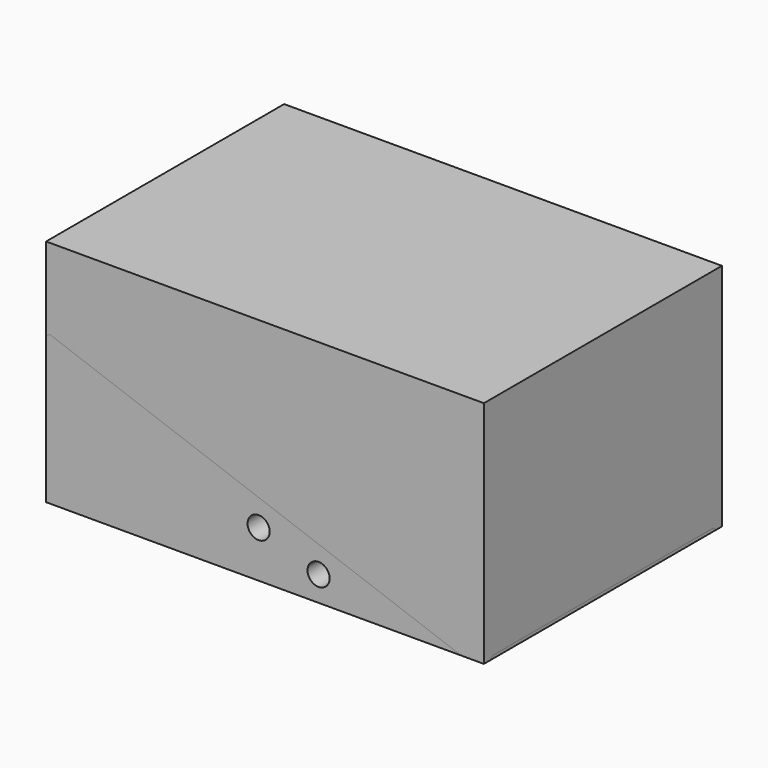
from build123d import *

# Parameters (mm, degrees)
F1_DEPTH      = 35
F1_DEPTH_BACK = 35
F14_W         = 103
F14_H         = 70
F15_DEPTH     = 54
F16_T1_DEPTH  = 122.3961453181
F16_T3_DEPTH  = 88.1090116667
F19_START     = 30
F19_DEPTH     = 5
F20_START     = -30
F20_DEPTH     = 5
F21_R         = 2.6
F22_DEPTH     = 5


# Not quite as in the source:
# - a fillet or chamfer that OpenCascade refuses, or shapes differently, is made with other operations: its cross-section is extruded or revolved along the edge and cut away or added
# - a feature names something its author has since deleted; it is built from what else it names


with BuildPart() as f1:
    # F0 (on Front) → F1 (new body, two sides)
    with BuildSketch(Plane.XZ) as f1_sk:
        Polygon((0, 38), (0, 0), (103, 0), (103, 0.7238095238), align=None)
    extrude(amount=F1_DEPTH)
    extrude(f1_sk.sketch, amount=-F1_DEPTH_BACK)

    # F3 (on offset) → F4 (revolve, cut)
    with BuildSketch(Plane(origin=(12.1597561954, 0, 33.5993263293), x_dir=(0.9403152653, 0, -0.3403045722), z_dir=(0.3403045722, 0, 0.9403152653))):
        with BuildLine():
            ThreePointArc((-3.1315737436, 0), (22.0684262564, -25.2), (47.2684262564, 0))
            Line((47.2684262564, 0), (-3.1315737436, 0))
        make_face()
    revolve(axis=Axis((32.9110342852, 0, 26.089339973), (0.9403152653, 0, -0.3403045722)), mode=Mode.SUBTRACT)

    # F3 (on offset) → F5 (revolve, cut)
    with BuildSketch(Plane(origin=(12.1597561954, 0, 33.5993263293), x_dir=(0.9403152653, 0, -0.3403045722), z_dir=(0.3403045722, 0, 0.9403152653))):
        with BuildLine():
            ThreePointArc((56.9684262564, -15), (62.0684262564, -20.1), (67.1684262564, -15))
            Line((67.1684262564, -15), (62.0684262564, -15))
            Line((62.0684262564, -15), (56.9684262564, -15))
        make_face()
    revolve(axis=Axis((68.1258409703, -15, 13.3449337441), (-0.9403152653, 0, 0.3403045722)), mode=Mode.SUBTRACT)

    # F3 (on offset) → F6 (revolve, cut)
    with BuildSketch(Plane(origin=(12.1597561954, 0, 33.5993263293), x_dir=(0.9403152653, 0, -0.3403045722), z_dir=(0.3403045722, 0, 0.9403152653))):
        with BuildLine():
            ThreePointArc((51.8684262564, 15), (62.0684262564, 4.8), (72.2684262564, 15))
            Line((72.2684262564, 15), (62.0684262564, 15))
            Line((62.0684262564, 15), (51.8684262564, 15))
        make_face()
    revolve(axis=Axis((65.7280370438, 15, 14.2127104032), (-0.9403152653, 0, 0.3403045722)), mode=Mode.SUBTRACT)

    # F3 (on offset) → F7 (revolve, cut)
    with BuildSketch(Plane(origin=(12.1597561954, 0, 33.5993263293), x_dir=(0.9403152653, 0, -0.3403045722), z_dir=(0.3403045722, 0, 0.9403152653))):
        with BuildLine():
            ThreePointArc((80.0684262564, -15), (82.0684262564, -17), (84.0684262564, -15))
            Line((84.0684262564, -15), (82.0684262564, -15))
            Line((82.0684262564, -15), (80.0684262564, -15))
        make_face()
    revolve(axis=Axis((88.3896349374, -15, 6.0113702131), (-0.9403152653, 0, 0.3403045722)), mode=Mode.SUBTRACT)

    # F3 (on offset) → F8 (revolve, cut)
    with BuildSketch(Plane(origin=(12.1597561954, 0, 33.5993263293), x_dir=(0.9403152653, 0, -0.3403045722), z_dir=(0.3403045722, 0, 0.9403152653))):
        with BuildLine():
            ThreePointArc((79.4684262564, 15), (82.0684262564, 12.4), (84.6684262564, 15))
            Line((84.6684262564, 15), (82.0684262564, 15))
            Line((82.0684262564, 15), (79.4684262564, 15))
        make_face()
    revolve(axis=Axis((88.1075403578, 15, 6.1134615848), (-0.9403152653, 0, 0.3403045722)), mode=Mode.SUBTRACT)

    # F16: chamfer of 2.5 on 3 edges, made by hand

    # F16_s2 → F16_t1 (cut)
    with BuildSketch(Plane(origin=(96.8857257323, 0, -35.0634055031), x_dir=(0, 1, 0), z_dir=(-0.9403152653, 0, 0.3403045722))):
        Polygon((-32.5, -35.7319800811), (-35, -33.2319800811), (-35, -35.7319800811), align=None)
        Polygon((32.5, -35.7319800811), (35, -33.2319800811), (35, -35.7319800811), align=None)
    extrude(amount=F16_T1_DEPTH, mode=Mode.SUBTRACT)

    # F16_s4 → F16_t3 (cut)
    with BuildSketch(Plane.XZ.offset(-44.0545058334)):
        Polygon((3.3507614305, 36.7873434823), (0, 34.4365553191), (0, 38), align=None)
    extrude(amount=F16_T3_DEPTH, mode=Mode.SUBTRACT)


with BuildPart() as f9:
    # F3 (on offset) → F9 (revolve)
    with BuildSketch(Plane(origin=(12.1597561954, 0, 33.5993263293), x_dir=(0.9403152653, 0, -0.3403045722), z_dir=(0.3403045722, 0, 0.9403152653))):
        with BuildLine():
            ThreePointArc((-3.1315737436, 0), (22.0684262564, -25.2), (47.2684262564, 0))
            Line((47.2684262564, 0), (-3.1315737436, 0))
        make_face()
    revolve(axis=Axis((32.9110342852, 0, 26.089339973), (0.9403152653, 0, -0.3403045722)))


with BuildPart() as f10:
    # F3 (on offset) → F10 (revolve)
    with BuildSketch(Plane(origin=(12.1597561954, 0, 33.5993263293), x_dir=(0.9403152653, 0, -0.3403045722), z_dir=(0.3403045722, 0, 0.9403152653))):
        with BuildLine():
            ThreePointArc((51.8684262564, 15), (62.0684262564, 4.8), (72.2684262564, 15))
            Line((72.2684262564, 15), (62.0684262564, 15))
            Line((62.0684262564, 15), (51.8684262564, 15))
        make_face()
    revolve(axis=Axis((65.7280370438, 15, 14.2127104032), (-0.9403152653, 0, 0.3403045722)))


with BuildPart() as f11:
    # F3 (on offset) → F11 (revolve)
    with BuildSketch(Plane(origin=(12.1597561954, 0, 33.5993263293), x_dir=(0.9403152653, 0, -0.3403045722), z_dir=(0.3403045722, 0, 0.9403152653))):
        with BuildLine():
            ThreePointArc((56.9684262564, -15), (62.0684262564, -20.1), (67.1684262564, -15))
            Line((67.1684262564, -15), (62.0684262564, -15))
            Line((62.0684262564, -15), (56.9684262564, -15))
        make_face()
    revolve(axis=Axis((68.1258409703, -15, 13.3449337441), (-0.9403152653, 0, 0.3403045722)))


with BuildPart() as f12:
    # F3 (on offset) → F12 (revolve)
    with BuildSketch(Plane(origin=(12.1597561954, 0, 33.5993263293), x_dir=(0.9403152653, 0, -0.3403045722), z_dir=(0.3403045722, 0, 0.9403152653))):
        with BuildLine():
            ThreePointArc((79.4684262564, 15), (82.0684262564, 12.4), (84.6684262564, 15))
            Line((84.6684262564, 15), (82.0684262564, 15))
            Line((82.0684262564, 15), (79.4684262564, 15))
        make_face()
    revolve(axis=Axis((88.1075403578, 15, 6.1134615848), (-0.9403152653, 0, 0.3403045722)))


with BuildPart() as f13:
    # F3 (on offset) → F13 (revolve)
    with BuildSketch(Plane(origin=(12.1597561954, 0, 33.5993263293), x_dir=(0.9403152653, 0, -0.3403045722), z_dir=(0.3403045722, 0, 0.9403152653))):
        with BuildLine():
            ThreePointArc((80.0684262564, -15), (82.0684262564, -17), (84.0684262564, -15))
            Line((84.0684262564, -15), (82.0684262564, -15))
            Line((82.0684262564, -15), (80.0684262564, -15))
        make_face()
    revolve(axis=Axis((88.3896349374, -15, 6.0113702131), (-0.9403152653, 0, 0.3403045722)))


with BuildPart() as f15:
    # F14 (on Top) → F15 (new body)
    with BuildSketch(Plane.XY):
        with Locations((51.5, 0)):
            Rectangle(F14_W, F14_H)
    extrude(amount=F15_DEPTH)

    # F17: cut F13, F12, F11, F10, F9, F1
    add(f13.part, mode=Mode.SUBTRACT)
    add(f12.part, mode=Mode.SUBTRACT)
    add(f11.part, mode=Mode.SUBTRACT)
    add(f10.part, mode=Mode.SUBTRACT)
    add(f9.part, mode=Mode.SUBTRACT)
    add(f1.part, mode=Mode.SUBTRACT)


with BuildPart() as f1_1:
    add(f1.part)

    # F18 (on Front) → F19 (cut)
    with BuildSketch(Plane.XZ.offset(F19_START)):
        with BuildLine():
            ThreePointArc((52.4448196898, 10.1152081123), (52.5609110872, 10.5508514685), (52.6, 11))
            ThreePointArc((52.6, 11), (47.4390889128, 11.4491485315), (52.4448196898, 10.1152081123))
        make_face()
        with BuildLine():
            ThreePointArc((66.7047289794, 5.895431417), (64.5538775108, 8.4563425042), (61.6599092896, 6.7802233047))
            ThreePointArc((61.6599092896, 6.7802233047), (63.6555804479, 3.3345203298), (66.7047289794, 5.895431417))
        make_face()
    extrude(amount=F19_DEPTH, mode=Mode.SUBTRACT)

    # F18 (on Front) → F20 (cut)
    with BuildSketch(Plane.XZ.offset(F20_START)):
        with BuildLine():
            ThreePointArc((52.4448196898, 10.1152081123), (52.5609110872, 10.5508514685), (52.6, 11))
            ThreePointArc((52.6, 11), (47.4390889128, 11.4491485315), (52.4448196898, 10.1152081123))
        make_face()
        with BuildLine():
            ThreePointArc((66.7047289794, 5.895431417), (64.5538775108, 8.4563425042), (61.6599092896, 6.7802233047))
            ThreePointArc((61.6599092896, 6.7802233047), (63.6555804479, 3.3345203298), (66.7047289794, 5.895431417))
        make_face()
    extrude(amount=-F20_DEPTH, mode=Mode.SUBTRACT)

    # F21 (on face) → F22 (cut)
    with BuildSketch(Plane(origin=(0, 0, 0), x_dir=(0, -1, 0), z_dir=(-1, 0, 0))):
        with Locations((-7.5, 29)):
            Circle(F21_R)
        with Locations((7.5, 29)):
            Circle(F21_R)
    extrude(amount=-F22_DEPTH, mode=Mode.SUBTRACT)


solid = Compound([f9.part, f10.part, f11.part, f12.part, f13.part, f15.part, f1_1.part])
